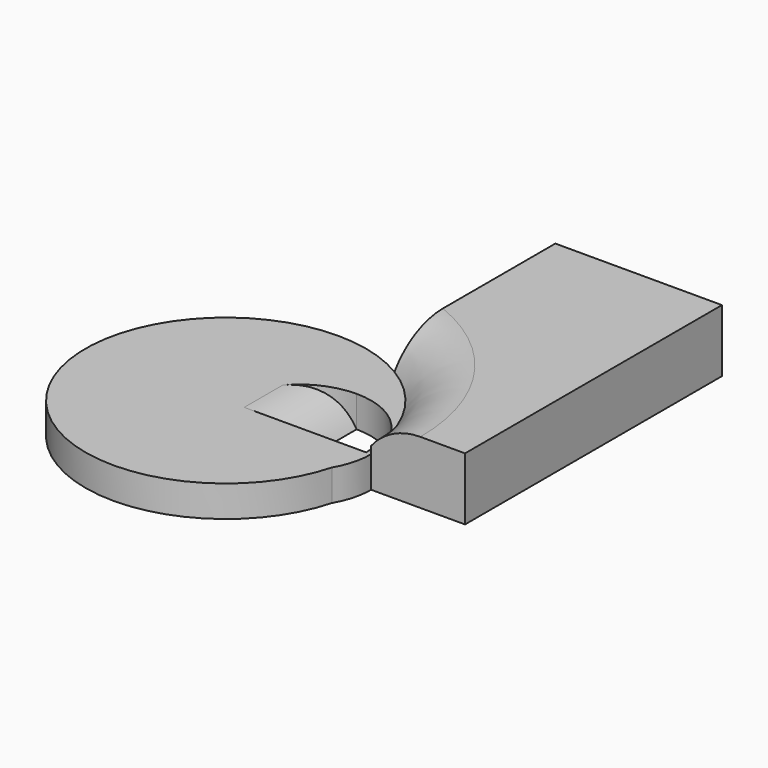
from build123d import *

# Parameters (mm, degrees)
F1_DEPTH     = 25.4
F2_DEPTH     = 12.7
F3_T4_DEPTH  = 139.4853841596
F3_S5_R      = 56.9586140596
F3_T6_DEPTH  = 72
F3_T11_DEPTH = 84.4927710193
F3_S12_R     = 29.500157879
F3_T13_DEPTH = 46
F3_T15_ANGLE = 154.3366921311


# Not quite as in the source:
# - a fillet or chamfer that OpenCascade refuses, or shapes differently, is made with other operations: its cross-section is extruded or revolved along the edge and cut away or added


with BuildPart() as f1:
    # F0 (on Top) → F1 (new body)
    with BuildSketch(Plane.XY):
        with BuildLine():
            ThreePointArc((-44.6654795557, 14.8543386834), (-41.6735799491, 7.6933988578), (-40.6527291, 0))
            Line((-40.6527291, 0), (-2.5527291, 0))
            Line((-2.5527291, 0), (-2.5527291, 130.3065121174))
            Line((-2.5527291, 130.3065121174), (-70.1528869789, 130.3065121174))
            Line((-70.1528869789, 130.3065121174), (-70.1528869789, 48.7239612584))
            ThreePointArc((-70.1528869789, 48.7239612584), (-54.141159867, 34.2483874097), (-44.6654795557, 14.8543386834))
        make_face()
    extrude(amount=F1_DEPTH)

    # F0 (on Top) → F2 (join)
    with BuildSketch(Plane.XY):
        with BuildLine():
            Line((-42.6944307983, 0), (-70.1528869789, 0))
            Line((-70.1528869789, 0), (-70.1528869789, 29.500157879))
            ThreePointArc((-70.1528869789, 29.500157879), (-95.730852606, -14.6978566215), (-44.6654795557, -14.8543386834))
            ThreePointArc((-44.6654795557, -14.8543386834), (-43.1893431296, -7.4922695314), (-42.6944307983, 0))
        make_face()
        with BuildLine():
            ThreePointArc((-44.6654795557, 14.8543386834), (-43.1893431296, 7.4922695314), (-42.6944307983, 0))
            Line((-42.6944307983, 0), (-40.6527291, 0))
            ThreePointArc((-40.6527291, 0), (-41.6735799491, 7.6933988578), (-44.6654795557, 14.8543386834))
        make_face()
        with BuildLine():
            Line((-40.6527291, 0), (-42.6944307983, 0))
            ThreePointArc((-42.6944307983, 0), (-43.1893431296, -7.4922695314), (-44.6654795557, -14.8543386834))
            ThreePointArc((-44.6654795557, -14.8543386834), (-41.6735799491, -7.6933988578), (-40.6527291, 0))
        make_face()
        with BuildLine():
            ThreePointArc((-44.6654795557, -14.8543386834), (-95.730852606, -14.6978566215), (-70.1528869789, 29.500157879))
            Line((-70.1528869789, 29.500157879), (-70.1528869789, 48.7239612584))
            ThreePointArc((-70.1528869789, 48.7239612584), (-152.5216924476, -21.1940986511), (-44.6654795557, -14.8543386834))
        make_face()
        with BuildLine():
            Line((-70.1528869789, 48.7239612584), (-70.1528869789, 29.500157879))
            ThreePointArc((-70.1528869789, 29.500157879), (-55.4550303574, 25.577965627), (-44.6654795557, 14.8543386834))
            ThreePointArc((-44.6654795557, 14.8543386834), (-54.141159867, 34.2483874097), (-70.1528869789, 48.7239612584))
        make_face()
        with BuildLine():
            ThreePointArc((-44.6654795557, 14.8543386834), (-41.6735799491, 7.6933988578), (-40.6527291, 0))
            Line((-40.6527291, 0), (-2.5527291, 0))
            Line((-2.5527291, 0), (-2.5527291, 130.3065121174))
            Line((-2.5527291, 130.3065121174), (-70.1528869789, 130.3065121174))
            Line((-70.1528869789, 130.3065121174), (-70.1528869789, 48.7239612584))
            ThreePointArc((-70.1528869789, 48.7239612584), (-54.141159867, 34.2483874097), (-44.6654795557, 14.8543386834))
        make_face()
    extrude(amount=F2_DEPTH)

    # F3: fillet of radius 25.4 on 2 edges, made by hand


with BuildPart() as f3_tool2:
    # F3_s3 → F3_t4 (new body)
    with BuildSketch(Plane.XZ.offset(54.9926131403)):
        with BuildLine():
            ThreePointArc((-92.1499322351, 12.7), (-79.4499322351, 9.2970452561), (-70.1528869789, 0))
            Line((-70.1528869789, 0), (-69.7129460738, 0.254))
            ThreePointArc((-69.7129460738, 0.254), (-69.6448869789, 6.35), (-69.6448869789, 12.7))
            Line((-69.6448869789, 12.7), (-70.1528869789, 13.208))
            Line((-70.1528869789, 13.208), (-92.1499322351, 13.208))
            Line((-92.1499322351, 13.208), (-92.1499322351, 12.7))
        make_face()
    extrude(amount=-F3_T4_DEPTH)

    # F3_s5 → F3_t6 (cut, symmetric)
    with BuildSketch(Plane.XY.offset(6.6)):
        with Locations((-99.6530448579, 0)):
            Circle(F3_S5_R)
    extrude(amount=F3_T6_DEPTH, both=True, mode=Mode.SUBTRACT)

    split(bisect_by=Plane.XZ, keep=Keep.TOP)


with BuildPart() as f1_1:
    add(f1.part)

    # F3_t1: cut F3_tool2
    add(f3_tool2.part, mode=Mode.SUBTRACT)


with BuildPart() as f3_tool9:
    # F3_s10 → F3_t11 (new body)
    with BuildSketch(Plane.XZ):
        with BuildLine():
            ThreePointArc((-92.1499322351, 12.7), (-79.4499322351, 9.2970452561), (-70.1528869789, 0))
            Line((-70.1528869789, 0), (-69.7129460738, 0.254))
            ThreePointArc((-69.7129460738, 0.254), (-69.6448869789, 6.35), (-69.6448869789, 12.7))
            Line((-69.6448869789, 12.7), (-70.1528869789, 13.208))
            Line((-70.1528869789, 13.208), (-92.1499322351, 13.208))
            Line((-92.1499322351, 13.208), (-92.1499322351, 12.7))
        make_face()
    extrude(amount=-F3_T11_DEPTH)

    # F3_s12 → F3_t13 (intersect, symmetric)
    with BuildSketch(Plane.XY.offset(6.6)):
        with Locations((-70.1528869789, 0)):
            Circle(F3_S12_R)
    extrude(amount=F3_T13_DEPTH, both=True, mode=Mode.INTERSECT)


with BuildPart() as f1_2:
    add(f1_1.part)

    # F3_t8: cut F3_tool9
    add(f3_tool9.part, mode=Mode.SUBTRACT)

    # F3_s14 → F3_t15 (revolve, cut)
    with BuildSketch(Plane(origin=(-82.9981282802, -37.1796571073, 0), x_dir=(0, 0, 1), z_dir=(-0.912617648, -0.4088141736, 0))):
        with BuildLine():
            ThreePointArc((25.4, 119.695236496), (21.9970452561, 106.995236496), (12.7, 97.6981912399))
            Line((12.7, 97.6981912399), (12.954, 97.2582503348))
            ThreePointArc((12.954, 97.2582503348), (19.05, 97.1901912399), (25.4, 97.1901912399))
            Line((25.4, 97.1901912399), (25.908, 97.6981912399))
            Line((25.908, 97.6981912399), (25.908, 119.695236496))
            Line((25.908, 119.695236496), (25.4, 119.695236496))
        make_face()
    revolve(axis=Axis((-99.6530448579, 0, 25.4), (0, 0, -1)), revolution_arc=F3_T15_ANGLE, mode=Mode.SUBTRACT)


solid = f1_2.part
